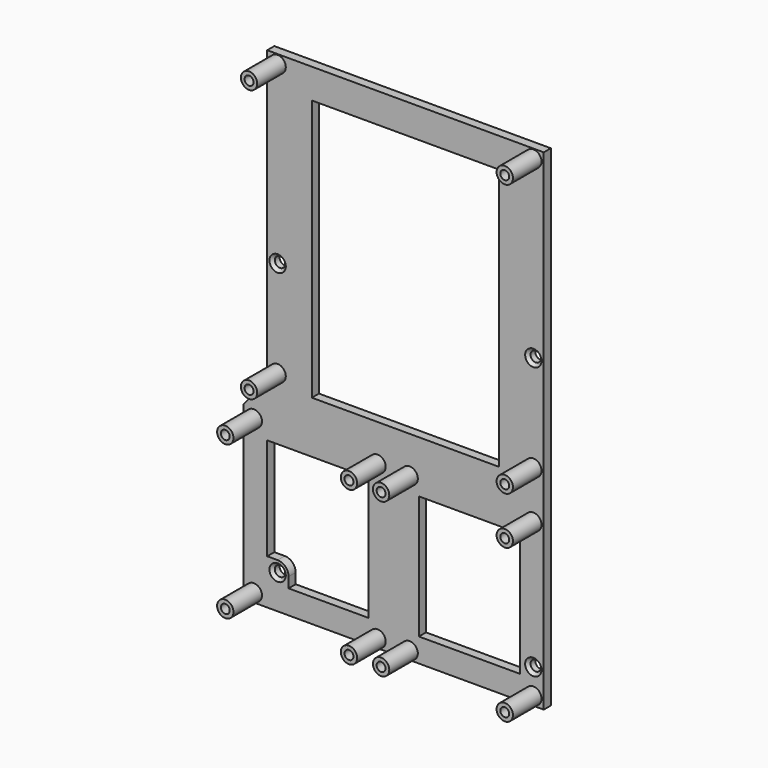
from build123d import *

# Parameters (mm, degrees)
F0_R     = 2.75
F0_R_2   = 1.5
F1_DEPTH = 15
F0_R_3   = 1.75
F0_W     = 63
F0_H     = 88
F0_W_2   = 101
F0_H_2   = 57.5
F0_W_3   = 34
F0_H_3   = 41.5
F2_DEPTH = 3
F3_SIZE  = 1


# Not quite as in the source:
# - ends of sketch curves that miss each other by under 0.0002 mm in the source are joined


with BuildPart() as f1:
    # F0 (on Front) → F1 (new body)
    with BuildSketch(Plane.XZ):
        with Locations((-89.5, 94.5)):
            Circle(F0_R)
        with Locations((-89.5, 94.5)):
            Circle(F0_R_2, mode=Mode.SUBTRACT)
    extrude(amount=F1_DEPTH)


with BuildPart() as f1b:
    # F0 (on Front) → F1, piece 2 (new body)
    with BuildSketch(Plane.XZ):
        with Locations((-3.5, 94.5)):
            Circle(F0_R)
        with Locations((-3.5, 94.5)):
            Circle(F0_R_2, mode=Mode.SUBTRACT)
    extrude(amount=F1_DEPTH)


with BuildPart() as f1c:
    # F0 (on Front) → F1, piece 3 (new body)
    with BuildSketch(Plane.XZ):
        with Locations((-89.5, 3)):
            Circle(F0_R)
        with Locations((-89.5, 3)):
            Circle(F0_R_2, mode=Mode.SUBTRACT)
    extrude(amount=F1_DEPTH)


with BuildPart() as f1d:
    # F0 (on Front) → F1, piece 4 (new body)
    with BuildSketch(Plane.XZ):
        with Locations((-3.5, 3)):
            Circle(F0_R)
        with Locations((-3.5, 3)):
            Circle(F0_R_2, mode=Mode.SUBTRACT)
    extrude(amount=F1_DEPTH)


with BuildPart() as f1e:
    # F0 (on Front) → F1, piece 5 (new body)
    with BuildSketch(Plane.XZ):
        with Locations((-3.5, -13)):
            Circle(F0_R)
        with Locations((-3.5, -13)):
            Circle(F0_R_2, mode=Mode.SUBTRACT)
    extrude(amount=F1_DEPTH)


with BuildPart() as f1f:
    # F0 (on Front) → F1, piece 6 (new body)
    with BuildSketch(Plane.XZ):
        with Locations((-45.0998449271, -12.8864128417)):
            Circle(F0_R)
        with Locations((-45.0998449271, -12.8864128417)):
            Circle(F0_R_2, mode=Mode.SUBTRACT)
    extrude(amount=F1_DEPTH)


with BuildPart() as f1g:
    # F0 (on Front) → F1, piece 7 (new body)
    with BuildSketch(Plane.XZ):
        with Locations((-55.9001550729, -12.8864128417)):
            Circle(F0_R)
        with Locations((-55.9001550729, -12.8864128417)):
            Circle(F0_R_2, mode=Mode.SUBTRACT)
    extrude(amount=F1_DEPTH)


with BuildPart() as f1h:
    # F0 (on Front) → F1, piece 8 (new body)
    with BuildSketch(Plane.XZ):
        with Locations((-97.5, -13)):
            Circle(F0_R)
        with Locations((-97.5, -13)):
            Circle(F0_R_2, mode=Mode.SUBTRACT)
    extrude(amount=F1_DEPTH)


with BuildPart() as f1i:
    # F0 (on Front) → F1, piece 9 (new body)
    with BuildSketch(Plane.XZ):
        with Locations((-97.5, -64.5)):
            Circle(F0_R)
        with Locations((-97.5, -64.5)):
            Circle(F0_R_2, mode=Mode.SUBTRACT)
    extrude(amount=F1_DEPTH)


with BuildPart() as f1j:
    # F0 (on Front) → F1, piece 10 (new body)
    with BuildSketch(Plane.XZ):
        with Locations((-55.9001550729, -64.6135871583)):
            Circle(F0_R)
        with Locations((-55.9001550729, -64.6135871583)):
            Circle(F0_R_2, mode=Mode.SUBTRACT)
    extrude(amount=F1_DEPTH)


with BuildPart() as f1k:
    # F0 (on Front) → F1, piece 11 (new body)
    with BuildSketch(Plane.XZ):
        with Locations((-45.0998449271, -64.6135871583)):
            Circle(F0_R)
        with Locations((-45.0998449271, -64.6135871583)):
            Circle(F0_R_2, mode=Mode.SUBTRACT)
    extrude(amount=F1_DEPTH)


with BuildPart() as f1l:
    # F0 (on Front) → F1, piece 12 (new body)
    with BuildSketch(Plane.XZ):
        with Locations((-3.5, -64.5)):
            Circle(F0_R)
        with Locations((-3.5, -64.5)):
            Circle(F0_R_2, mode=Mode.SUBTRACT)
    extrude(amount=F1_DEPTH)


with BuildPart() as f2:
    # F0 (on Front) → F2 (new body)
    with BuildSketch(Plane.XZ):
        Polygon((0, 97.5), (-93, 97.5), (-93, 0), (-101, -10), (0, -10), (0, 0), align=None)
        with Locations((-89.5, 3)):
            Circle(F0_R, mode=Mode.SUBTRACT)
        with Locations((-3.5, 3)):
            Circle(F0_R, mode=Mode.SUBTRACT)
        with Locations((-89.5, 35.5)):
            Circle(F0_R_3, mode=Mode.SUBTRACT)
        with Locations((-89.5, 94.5)):
            Circle(F0_R, mode=Mode.SUBTRACT)
        with Locations((-46.5, 43.5)):
            Rectangle(F0_W, F0_H, mode=Mode.SUBTRACT)
        with Locations((-3.5, 35.5)):
            Circle(F0_R_3, mode=Mode.SUBTRACT)
        with Locations((-3.5, 94.5)):
            Circle(F0_R, mode=Mode.SUBTRACT)
        with Locations((-50.5, -38.75)):
            Rectangle(F0_W_2, F0_H_2)
        with Locations((-97.5, -64.5)):
            Circle(F0_R, mode=Mode.SUBTRACT)
        with Locations((-89.5, -56)):
            Circle(F0_R_3, mode=Mode.SUBTRACT)
        with BuildLine():
            Line((-93, -52.3246), (-93, -18))
            Line((-93, -18), (-59, -18))
            Line((-59, -18), (-59, -59.5))
            Line((-59, -59.5), (-85.824604243, -59.5))
            Line((-85.824604243, -59.5), (-85.824604243, -56))
            ThreePointArc((-85.824604243, -56), (-86.9011027367, -53.4011027367), (-89.5, -52.324604243))
            Line((-89.5, -52.324604243), (-93, -52.3246))
        make_face(mode=Mode.SUBTRACT)
        with Locations((-55.9001550729, -64.6135871583)):
            Circle(F0_R, mode=Mode.SUBTRACT)
        with Locations((-97.5, -13)):
            Circle(F0_R, mode=Mode.SUBTRACT)
        with Locations((-55.9001550729, -12.8864128417)):
            Circle(F0_R, mode=Mode.SUBTRACT)
        with Locations((-45.0998449271, -64.6135871583)):
            Circle(F0_R, mode=Mode.SUBTRACT)
        with Locations((-3.5, -64.5)):
            Circle(F0_R, mode=Mode.SUBTRACT)
        with Locations((-3.5, -56)):
            Circle(F0_R_3, mode=Mode.SUBTRACT)
        with Locations((-25, -38.75)):
            Rectangle(F0_W_3, F0_H_3, mode=Mode.SUBTRACT)
        with Locations((-45.0998449271, -12.8864128417)):
            Circle(F0_R, mode=Mode.SUBTRACT)
        with Locations((-3.5, -13)):
            Circle(F0_R, mode=Mode.SUBTRACT)
    extrude(amount=F2_DEPTH)

    # F3
    f3_edges = [f2.edges().sort_by_distance(p)[0] for p in [
        (-91.25, -3, 35.5),
        (-5.25, -3, 35.5),
        (-5.25, -3, -56),
        (-91.25, -3, -56),
    ]]
    chamfer(f3_edges, length=F3_SIZE)


solid = Compound([f1.part, f1b.part, f1c.part, f1d.part, f1e.part, f1f.part, f1g.part, f1h.part, f1i.part, f1j.part, f1k.part, f1l.part, f2.part])
